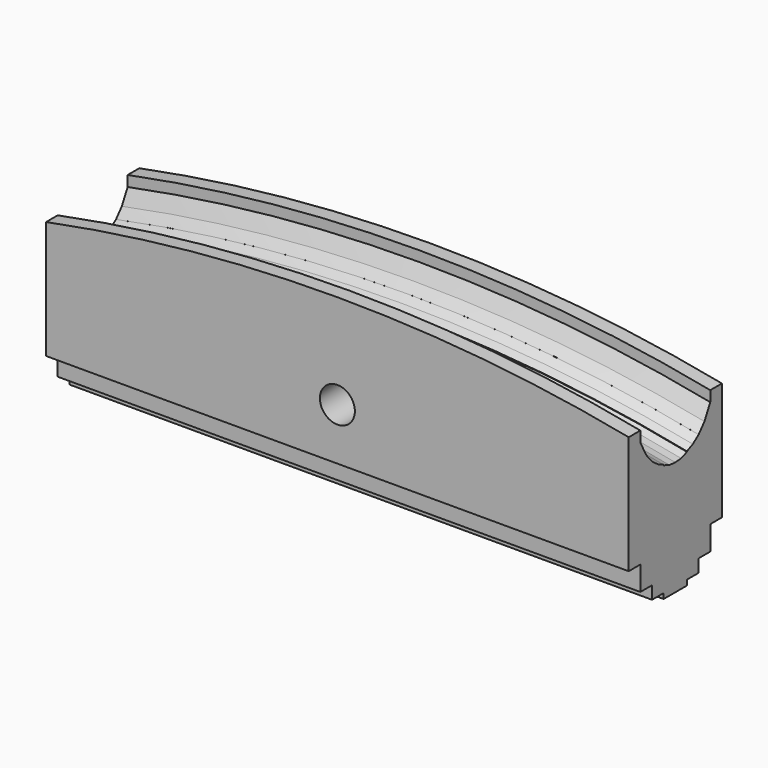
from build123d import *

# Parameters (mm, degrees)
F0_R      = 6
F1_DEPTH  = 5
F2_R      = 6
F3_DEPTH  = 5
F4_R      = 6
F5_DEPTH  = 5
F6_R      = 6
F7_DEPTH  = 5
F8_SIZE2  = 0.2055374144
F8_SIZE   = 2.5
F9_SIZE2  = 1.149871526
F9_SIZE   = 2.5
F10_SIZE2 = 2.8860789389
F10_SIZE  = 2.5
F11_SIZE2 = 0.909916
F11_SIZE  = 2.49999
F12_SIZE2 = 1.809688
F12_SIZE  = 2.49999
F13_SIZE2 = 4.721668
F13_SIZE  = 2.49999


# Not quite as in the source:
# - a fillet or chamfer is up to 0.001 mm smaller than in the source, because OpenCascade refuses the exact size


with BuildPart() as f1:
    # F0 (on Front) → F1 (new body)
    with BuildSketch(Plane.XZ):
        with BuildLine():
            Line((-100, 7.1879485566), (-100, -32.29))
            Line((-100, -32.29), (100, -32.29))
            Line((100, -32.29), (100, 7.1879485566))
            ThreePointArc((100, 7.1879485566), (0, 17.29), (-100, 7.1879485566))
        make_face()
        Circle(F0_R, mode=Mode.SUBTRACT)
    extrude(amount=F1_DEPTH)

    # F2 (on face) → F3 (join)
    with BuildSketch(Plane.XZ.offset(5)):
        with BuildLine():
            Line((-100, -30.49), (100, -30.49))
            Line((100, -30.49), (100, 9.4535179491))
            ThreePointArc((100, 9.4535179491), (0, 19.51), (-100, 9.4535179491))
            Line((-100, 9.4535179491), (-100, -30.49))
        make_face()
        Circle(F2_R, mode=Mode.SUBTRACT)
    extrude(amount=F3_DEPTH)

    # F4 (on face) → F5 (join)
    with BuildSketch(Plane.XZ.offset(10)):
        with BuildLine():
            Line((-100, -26.09), (100, -26.09))
            Line((100, -26.09), (100, 14.2486365081))
            ThreePointArc((100, 14.2486365081), (0, 24.21), (-100, 14.2486365081))
            Line((-100, 14.2486365081), (-100, -26.09))
        make_face()
        Circle(F4_R, mode=Mode.SUBTRACT)
    extrude(amount=F5_DEPTH)

    # F6 (on face) → F7 (join)
    with BuildSketch(Plane.XZ.offset(15)):
        with BuildLine():
            Line((-100, -17.79), (100, -17.79))
            Line((100, -17.79), (100, 22.7020537739))
            ThreePointArc((100, 22.7020537739), (0, 32.5), (-100, 22.7020537739))
            Line((-100, 22.7020537739), (-100, -17.79))
        make_face()
        Circle(F6_R, mode=Mode.SUBTRACT)
    extrude(amount=F7_DEPTH)

    # F8
    f8_edges = [f1.edges().sort_by_distance(p)[0] for p in [
        (0, 0, 17.29),
    ]]
    f8_side = f1.faces().sort_by_distance((0, -2.5, 17.29))[0]
    chamfer(f8_edges, length=F8_SIZE, length2=F8_SIZE2, reference=f8_side)

    # F9
    f9_edges = [f1.edges().sort_by_distance(p)[0] for p in [
        (0, -5, 19.51),
    ]]
    f9_side = f1.faces().sort_by_distance((0, -7.5, 19.51))[0]
    chamfer(f9_edges, length=F9_SIZE, length2=F9_SIZE2, reference=f9_side)

    # F10
    f10_edges = [f1.edges().sort_by_distance(p)[0] for p in [
        (0, -10, 24.21),
    ]]
    f10_side = f1.faces().sort_by_distance((0, -12.5, 24.21))[0]
    chamfer(f10_edges, length=F10_SIZE, length2=F10_SIZE2, reference=f10_side)

    # F11 (size 2.5 and 0.9099255857 in the source; OpenCascade refuses exactly that, so slightly less here)
    f11_edges = [f1.edges().sort_by_distance(p)[0] for p in [
        (0, -5, 17.29),
    ]]
    f11_side = f1.faces().sort_by_distance((0, -3.75, 17.29))[0]
    chamfer(f11_edges, length=F11_SIZE, length2=F11_SIZE2, reference=f11_side)

    # F12 (size 2.5 and 1.8096981916 in the source; OpenCascade refuses exactly that, so slightly less here)
    f12_edges = [f1.edges().sort_by_distance(p)[0] for p in [
        (0, -10, 19.51),
    ]]
    f12_side = f1.faces().sort_by_distance((0, -8.75, 19.51))[0]
    chamfer(f12_edges, length=F12_SIZE, length2=F12_SIZE2, reference=f12_side)

    # F13 (size 2.5 and 4.7216783541 in the source; OpenCascade refuses exactly that, so slightly less here)
    f13_edges = [f1.edges().sort_by_distance(p)[0] for p in [
        (0, -15, 24.21),
    ]]
    f13_side = f1.faces().sort_by_distance((0, -13.75, 24.21))[0]
    chamfer(f13_edges, length=F13_SIZE, length2=F13_SIZE2, reference=f13_side)

    # F14: F1 across plane


with BuildPart() as f1_1:
    add(f1.part)
    add(f1.part.mirror(Plane.XZ))


solid = f1_1.part
